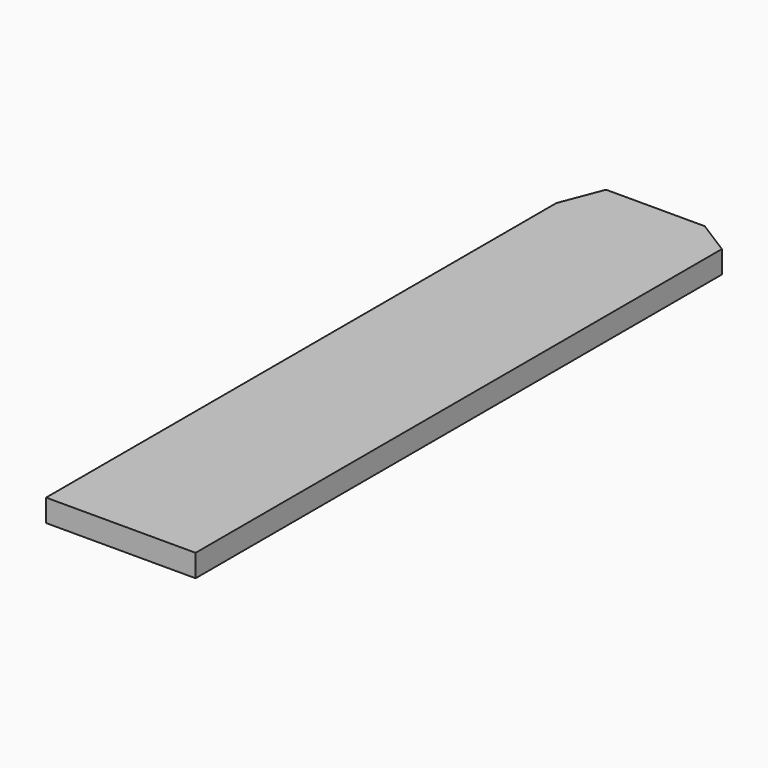
from build123d import *

# Parameters (mm, degrees)
F1_DEPTH = 19.05


# Not quite as in the source:
# - a feature names something its author has since deleted; it is built from what else it names


with BuildPart() as f1:
    # F0 (on Top) → F1 (new body)
    with BuildSketch(Plane.XY):
        Polygon((-35.3171963468, 328.1483577974), (-35.3171963468, -213.6605507338), (91.6828036532, -213.6605507338), (91.6828036532, 345.1394492662), (62.3207635859, 363.6657913806), (-21.5287261029, 363.6657913806), align=None)
    extrude(amount=F1_DEPTH)


solid = f1.part
